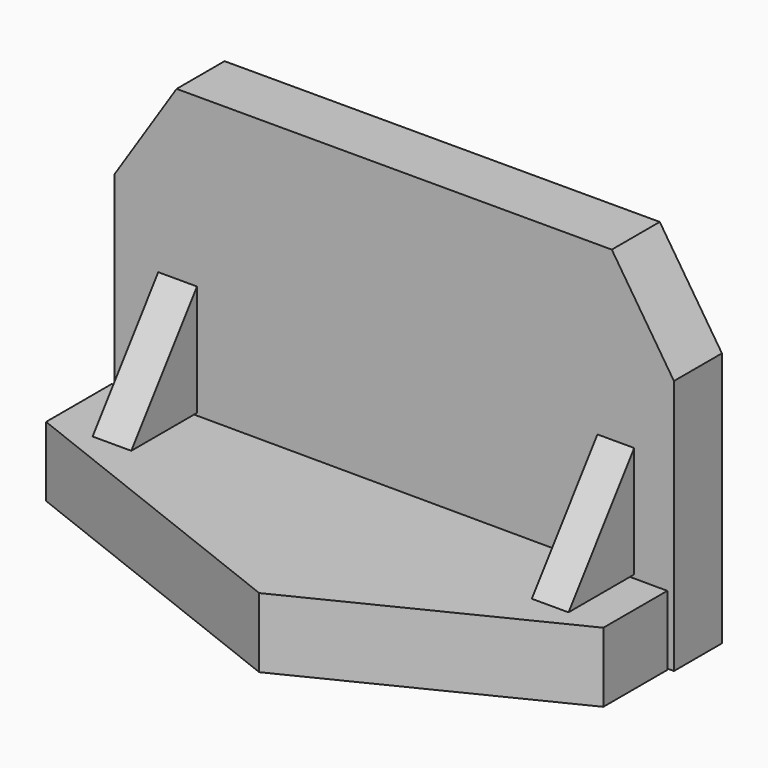
from build123d import *

# Parameters (mm, degrees)
F1_DEPTH = 7.874
F3_DEPTH = 9.144
F5_DEPTH = 27.432
F6_DEPTH = 22.606
F7_DEPTH = 35.052
F8_DEPTH = 29.972


with BuildPart() as f1:
    # F0 (on Front) → F1 (new body)
    with BuildSketch(Plane.XZ):
        Polygon((24.4839340448, 36.5801639855), (-32.6452478766, 36.5801639855), (-40.8065579832, 24.0467209369), (-40.8065579832, -9.472951293), (32.6452441514, -9.472951293), (32.6452441514, 24.0467209369), align=None)
    extrude(amount=F1_DEPTH)


with BuildPart() as f3:
    # F2 (on Top) → F3 (new body)
    with BuildSketch(Plane.XY):
        Polygon((32.3537737131, -8.5985241458), (-40.8065579832, -8.3070490509), (-40.8065579832, -19.0916396677), (0, -35.1227857172), (32.3537737131, -19.0916396677), align=None)
    extrude(amount=-F3_DEPTH)


with BuildPart() as f5:
    # F4 (on Right) → F5 (new body)
    with BuildSketch(Plane.YZ):
        Polygon((-18.6544265598, 0), (-7.5783613138, 0), (-7.5783613138, 15.0109836832), align=None)
    extrude(amount=F5_DEPTH)

    # F6 (cut): a face of the model
    f6_faces = [f5.faces().sort_by_distance(p)[0] for p in [
        (0, -11.2703830625, 5.0036612277),
    ]]
    extrude(f6_faces, amount=-F6_DEPTH, mode=Mode.SUBTRACT)


with BuildPart() as f7:
    # F4 (on Right) → F7 (new body)
    with BuildSketch(Plane.YZ):
        Polygon((-18.6544265598, 0), (-7.5783613138, 0), (-7.5783613138, 15.0109836832), align=None)
    extrude(amount=-F7_DEPTH)

    # F8 (cut): a face of the model
    f8_faces = [f7.faces().sort_by_distance(p)[0] for p in [
        (0, -11.2703830625, 5.0036612277),
    ]]
    extrude(f8_faces, amount=-F8_DEPTH, mode=Mode.SUBTRACT)


solid = Compound([f1.part, f3.part, f5.part, f7.part])
